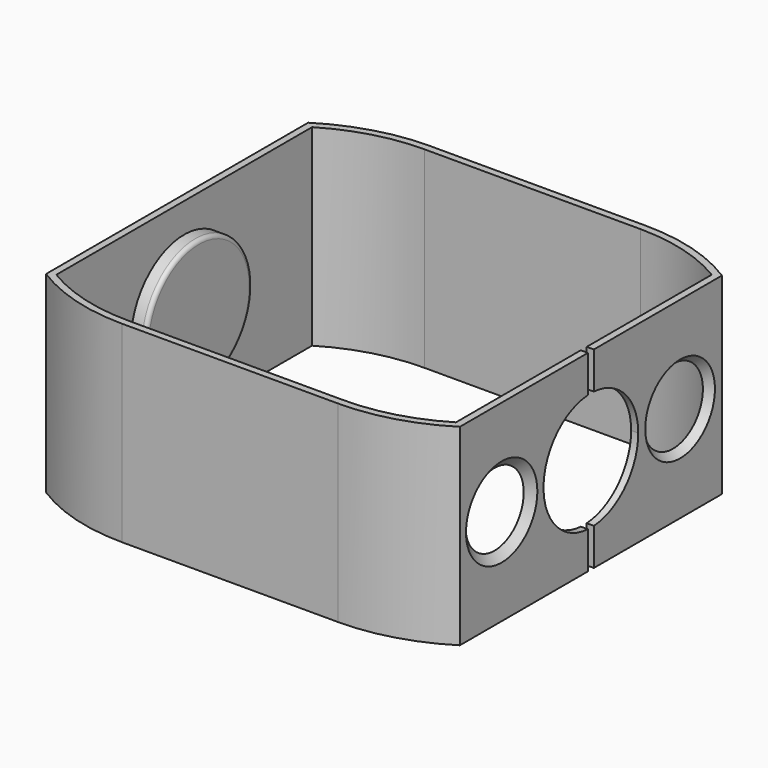
from build123d import *

# Parameters (mm, degrees)
F1_DEPTH = 10.31875
F2_R     = 3.90906
F3_DEPTH = 25.4
F4_DEPTH = 25.4
F6_R     = 7.14375
F7_DEPTH = 2.3495
F8_R     = 6.38175
F9_DEPTH = 1.5875
F10_R    = 0.4064


# Not quite as in the source:
# - a fillet or chamfer that OpenCascade refuses, or shapes differently, is made with other operations: its cross-section is extruded or revolved along the edge and cut away or added


with BuildPart() as f1:
    # F0 (on Top) → F1 (new body, symmetric)
    with BuildSketch(Plane.XY):
        with BuildLine():
            Line((0, 20.6466445854), (-11.58875, 20.6466445854))
            ThreePointArc((-11.58875, 20.6466445854), (-17.1096965819, 19.861848606), (-22.19325, 17.5696355848))
            Line((-22.19325, 17.5696355848), (-22.19325, -17.5696355848))
            ThreePointArc((-22.19325, -17.5696355848), (-17.1096965819, -19.861848606), (-11.58875, -20.6466445854))
            Line((-11.58875, -20.6466445854), (0, -20.6466445854))
            Line((0, -20.6466445854), (11.58875, -20.6466445854))
            ThreePointArc((11.58875, -20.6466445854), (17.1096965819, -19.861848606), (22.19325, -17.5696355848))
            Line((22.19325, -17.5696355848), (22.19325, 17.5696355848))
            ThreePointArc((22.19325, 17.5696355848), (17.1096965819, 19.861848606), (11.58875, 20.6466445854))
            Line((11.58875, 20.6466445854), (0, 20.6466445854))
        make_face()
        with BuildLine():
            ThreePointArc((11.58875, 19.8846445854), (16.6970877606, 19.1869573913), (21.43125, 17.145))
            Line((21.43125, 17.145), (21.43125, -17.145))
            ThreePointArc((21.43125, -17.145), (16.6970877606, -19.1869573913), (11.58875, -19.8846445854))
            Line((11.58875, -19.8846445854), (0, -19.8846445854))
            Line((0, -19.8846445854), (-11.58875, -19.8846445854))
            ThreePointArc((-11.58875, -19.8846445854), (-16.6970877606, -19.1869573913), (-21.43125, -17.145))
            Line((-21.43125, -17.145), (-21.43125, 17.145))
            ThreePointArc((-21.43125, 17.145), (-16.6970877606, 19.1869573913), (-11.58875, 19.8846445854))
            Line((-11.58875, 19.8846445854), (0, 19.8846445854))
            Line((0, 19.8846445854), (11.58875, 19.8846445854))
        make_face(mode=Mode.SUBTRACT)
    extrude(amount=F1_DEPTH, both=True)

    # F2 (on face) → F3 (cut)
    with BuildSketch(Plane.YZ.offset(22.19325)):
        with BuildLine():
            ThreePointArc((0.396875, -6.3375855209), (4.6283180665, -4.3475478002), (6.35, 0))
            ThreePointArc((6.35, 0), (4.6283180665, 4.3475478002), (0.396875, 6.3375855209))
            Line((0.396875, 6.3375855209), (0.396875, -6.3375855209))
        make_face()
        with BuildLine():
            Line((0.396875, -6.3375855209), (0.396875, 6.3375855209))
            ThreePointArc((0.396875, 6.3375855209), (0, 6.35), (-0.396875, 6.3375855209))
            Line((-0.396875, 6.3375855209), (-0.396875, -6.3375855209))
            ThreePointArc((-0.396875, -6.3375855209), (0, -6.35), (0.396875, -6.3375855209))
        make_face()
        with BuildLine():
            ThreePointArc((-0.396875, 6.3375855209), (0, 6.35), (0.396875, 6.3375855209))
            Line((0.396875, 6.3375855209), (0.396875, 16.235569492))
            Line((0.396875, 16.235569492), (-0.396875, 16.235569492))
            Line((-0.396875, 16.235569492), (-0.396875, 6.3375855209))
        make_face()
        with BuildLine():
            Line((0.396875, -16.235569492), (0.396875, -6.3375855209))
            ThreePointArc((0.396875, -6.3375855209), (0, -6.35), (-0.396875, -6.3375855209))
            Line((-0.396875, -6.3375855209), (-0.396875, -16.235569492))
            Line((-0.396875, -16.235569492), (0.396875, -16.235569492))
        make_face()
        with BuildLine():
            Line((-0.396875, -6.3375855209), (-0.396875, 6.3375855209))
            ThreePointArc((-0.396875, 6.3375855209), (-6.35, 0), (-0.396875, -6.3375855209))
        make_face()
        with Locations((-11.9634, 0)):
            Circle(F2_R)
        with Locations((11.9634, 0)):
            Circle(F2_R)
    extrude(amount=-F3_DEPTH, mode=Mode.SUBTRACT)

    # F2 (on face) → F4 (cut)
    with BuildSketch(Plane.YZ.offset(22.19325)):
        with BuildLine():
            ThreePointArc((0.396875, -6.3375855209), (4.6283180665, -4.3475478002), (6.35, 0))
            ThreePointArc((6.35, 0), (4.6283180665, 4.3475478002), (0.396875, 6.3375855209))
            Line((0.396875, 6.3375855209), (0.396875, -6.3375855209))
        make_face()
        with BuildLine():
            Line((0.396875, -6.3375855209), (0.396875, 6.3375855209))
            ThreePointArc((0.396875, 6.3375855209), (0, 6.35), (-0.396875, 6.3375855209))
            Line((-0.396875, 6.3375855209), (-0.396875, -6.3375855209))
            ThreePointArc((-0.396875, -6.3375855209), (0, -6.35), (0.396875, -6.3375855209))
        make_face()
        with BuildLine():
            ThreePointArc((-0.396875, 6.3375855209), (0, 6.35), (0.396875, 6.3375855209))
            Line((0.396875, 6.3375855209), (0.396875, 16.235569492))
            Line((0.396875, 16.235569492), (-0.396875, 16.235569492))
            Line((-0.396875, 16.235569492), (-0.396875, 6.3375855209))
        make_face()
        with BuildLine():
            Line((0.396875, -16.235569492), (0.396875, -6.3375855209))
            ThreePointArc((0.396875, -6.3375855209), (0, -6.35), (-0.396875, -6.3375855209))
            Line((-0.396875, -6.3375855209), (-0.396875, -16.235569492))
            Line((-0.396875, -16.235569492), (0.396875, -16.235569492))
        make_face()
        with BuildLine():
            Line((-0.396875, -6.3375855209), (-0.396875, 6.3375855209))
            ThreePointArc((-0.396875, 6.3375855209), (-6.35, 0), (-0.396875, -6.3375855209))
        make_face()
        with Locations((-11.9634, 0)):
            Circle(F2_R)
        with Locations((11.9634, 0)):
            Circle(F2_R)
    extrude(amount=-F4_DEPTH, mode=Mode.SUBTRACT)

    # F5: chamfer of 0.762 x 0.8765807263 on 2 edges, made by hand

    # F5_s1 → F5_t2 (revolve, cut)
    with BuildSketch(Plane.XY):
        Polygon((22.19325, -7.1777592737), (21.43125, -8.05434), (22.19325, -8.05434), align=None)
    revolve(axis=Axis((22.19325, -11.9634, 0), (1, 0, 0)), mode=Mode.SUBTRACT)

    # F5_s3 → F5_t4 (revolve, cut)
    with BuildSketch(Plane.XY):
        Polygon((22.19325, 16.63446), (21.3166692737, 15.87246), (22.19325, 15.87246), align=None)
    revolve(axis=Axis((22.19325, 11.9634, 0), (1, 0, 0)), mode=Mode.SUBTRACT)

    # F6 (on face) → F7 (join)
    with BuildSketch(Plane(origin=(-22.19325, 0, 0), x_dir=(0, -1, 0), z_dir=(-1, 0, 0))):
        Circle(F6_R)
    extrude(amount=-F7_DEPTH)

    # F8 (on face) → F9 (cut)
    with BuildSketch(Plane(origin=(-22.19325, 0, 0), x_dir=(0, -1, 0), z_dir=(-1, 0, 0))):
        Circle(F8_R)
    extrude(amount=-F9_DEPTH, mode=Mode.SUBTRACT)

    # F10
    f10_edges = [f1.edges().sort_by_distance(p)[0] for p in [
        (-22.19325, 6.38175, 0),
        (-20.60575, 6.38175, 0),
        (-19.84375, 7.14375, 0),
    ]]
    fillet(f10_edges, radius=F10_R)


solid = f1.part
